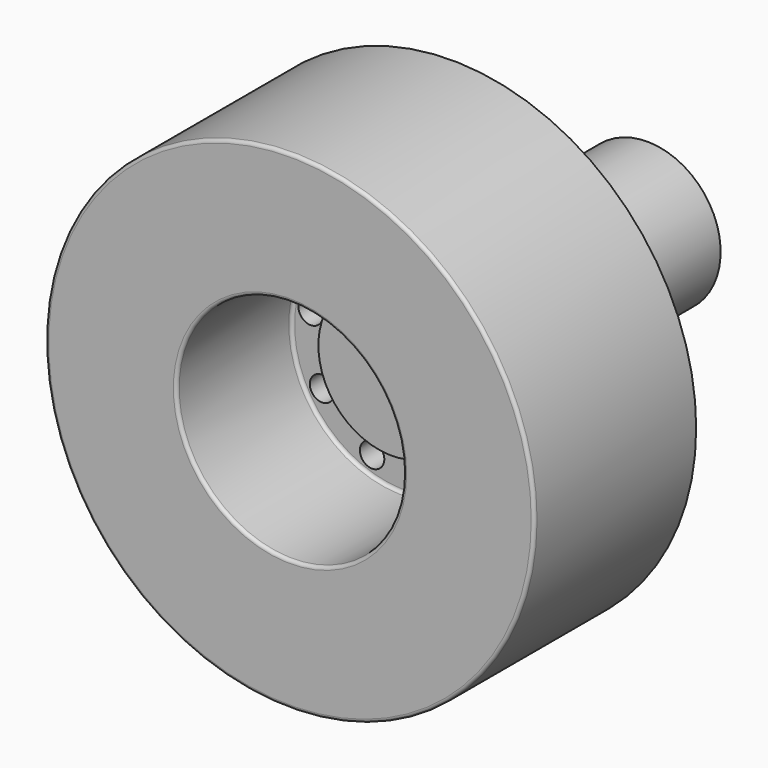
from build123d import *

# Parameters (mm, degrees)
F0_R      = 19.05
F1_DEPTH  = 15.748
F3_R      = 8.8392
F4_DEPTH  = 11.176
F5_R      = 0.254
F6_R      = 0.9525
F7_DEPTH  = 25.4
F8_R      = 5.715
F9_DEPTH  = 1.27
F11_R     = 18.0989194231
F11_R_2   = 11.2988088197
F12_DEPTH = 14.224
F10_R     = 5.715
F13_DEPTH = 19.05
F14_T     = 3.175


# Not quite as in the source:
# - a feature of the source that left no trace in its solid (it failed there, or was rolled back) is left out
# - a shell that OpenCascade refuses in one call is made with other operations: the cavity is built on its own and cut out


with BuildPart() as f1:
    # F0 (on Front) → F1 (new body)
    with BuildSketch(Plane.XZ):
        Circle(F0_R)
    extrude(amount=F1_DEPTH)

    # F3 (on face) → F4 (cut)
    with BuildSketch(Plane.XZ.offset(15.748)):
        Circle(F3_R)
    extrude(amount=-F4_DEPTH, mode=Mode.SUBTRACT)

    # F5
    f5_edges = [f1.edges().sort_by_distance(p)[0] for p in [
        (-8.8392, -15.748, 0),
        (8.8392, -10.16, 0),
        (-8.8392, -4.572, 0),
        (-19.05, -15.748, 0),
    ]]
    fillet(f5_edges, radius=F5_R)

    # F6 (on face) → F7 (cut)
    with BuildSketch(Plane.XZ.offset(4.572)):
        with Locations((0, 7.4422)):
            Circle(F6_R)
        with Locations((4.7837539488, 5.7010559546)):
            Circle(F6_R)
        with Locations((7.3291362595, 1.2923244678)):
            Circle(F6_R)
        with Locations((6.44513426, -3.7211)):
            Circle(F6_R)
        with Locations((2.5453823107, -6.9933804224)):
            Circle(F6_R)
        with Locations((-2.5453823107, -6.9933804224)):
            Circle(F6_R)
        with Locations((-6.44513426, -3.7211)):
            Circle(F6_R)
        with Locations((-7.3291362595, 1.2923244678)):
            Circle(F6_R)
        with Locations((-4.7837539488, 5.7010559546)):
            Circle(F6_R)
    extrude(amount=-F7_DEPTH, mode=Mode.SUBTRACT)

    # F8 (on face) → F9 (join)
    with BuildSketch(Plane.XZ.offset(4.572)):
        Circle(F8_R)
    extrude(amount=F9_DEPTH)

    # F11 (on face) → F12 (cut)
    with BuildSketch(Plane(origin=(0, 0, 0), x_dir=(-1, 0, 0), z_dir=(0, 1, 0))):
        Circle(F11_R)
        Circle(F11_R_2, mode=Mode.SUBTRACT)
    extrude(amount=-F12_DEPTH, mode=Mode.SUBTRACT)

    # F10 (on face) → F13 (join)
    with BuildSketch(Plane(origin=(0, 0, 0), x_dir=(-1, 0, 0), z_dir=(0, 1, 0))):
        Circle(F10_R)
    extrude(amount=F13_DEPTH)

    # F14: shell of thickness 3.175, made by hand


with BuildPart() as f14_core1:
    # F14_t2: copy of F1
    add(f1.part)

    # the walls: a layer under each face that stays
    f14_faces = [f14_core1.faces().sort_by_distance(p)[0] for p in [
        (-19.05, -7.747, 0),
        (-17.78, 0, -5.08),
        (-12.5306666667, -15.748, -12.5306666667),
        (18.0989194231, -7.112, 0),
        (12.065946282, -14.224, -12.065946282),
        (-8.8392, -10.16, 0),
        (11.2988088197, -7.112, 0),
        (-8.7648051224, -4.6463948776, 0),
        (-7.5325392131, 0, -7.5325392131),
        (-5.7234666667, -4.572, -5.7234666667),
        (-3.4978823107, -2.286, -6.9933804224),
        (-7.39763426, -2.286, -3.7211),
        (1.5928823107, -2.286, -6.9933804224),
        (5.715, 9.525, 0),
        (5.49263426, -2.286, -3.7211),
        (-8.2816362595, -2.286, 1.2923244678),
        (-5.7362539488, -2.286, 5.7010559546),
        (-0.9525, -2.286, 7.4422),
        (6.3766362595, -2.286, 1.2923244678),
        (3.8312539488, -2.286, 5.7010559546),
        (-5.715, -5.207, 0),
        (0, -5.842, 0),
    ]]
    thicken(f14_faces, amount=-F14_T, mode=Mode.SUBTRACT)

    # F14_s3 → F14_t4 (revolve, cut)
    with BuildSketch(Plane.XY):
        Polygon((-18.0671694231, -14.19225), (-21.2739194231, -14.224), (-21.2739194231, -17.399), (-18.0989194231, -17.399), align=None)
    revolve(axis=Axis((0, -14.224, 0), (0, 1, 0)), mode=Mode.SUBTRACT)

    # F14_s5 → F14_t6 (revolve, cut)
    with BuildSketch(Plane.XY):
        Polygon((-11.3305588197, -14.19225), (-11.2988088197, -17.399), (-8.1238088197, -17.399), (-8.1238088197, -14.224), align=None)
    revolve(axis=Axis((0, -14.224, 0), (0, 1, 0)), mode=Mode.SUBTRACT)

    # F14_s7 → F14_t8 (revolve, cut)
    with BuildSketch(Plane.XY):
        Polygon((-5.74675, 0.03175), (-5.715, -3.175), (-2.54, -3.175), (-2.54, 0), align=None)
    revolve(axis=Axis((0, 0, 0), (0, 1, 0)), mode=Mode.SUBTRACT)

    # F14_s9 → F14_t10 (revolve, cut)
    with BuildSketch(Plane.XY):
        Polygon((5.74675, -4.60375), (5.715, -1.397), (2.54, -1.397), (2.54, -4.572), align=None)
    revolve(axis=Axis((0, -4.572, 0), (0, -1, 0)), mode=Mode.SUBTRACT)


with BuildPart() as f1_1:
    add(f1.part)

    # what is left inside the walls is the cavity
    f14_cavity = [f14_core1.part.solids().sort_by_distance(p)[0] for p in [
        (2.50825, 4.572, 0),
    ]]
    add(f14_cavity, mode=Mode.SUBTRACT)


solid = f1_1.part
